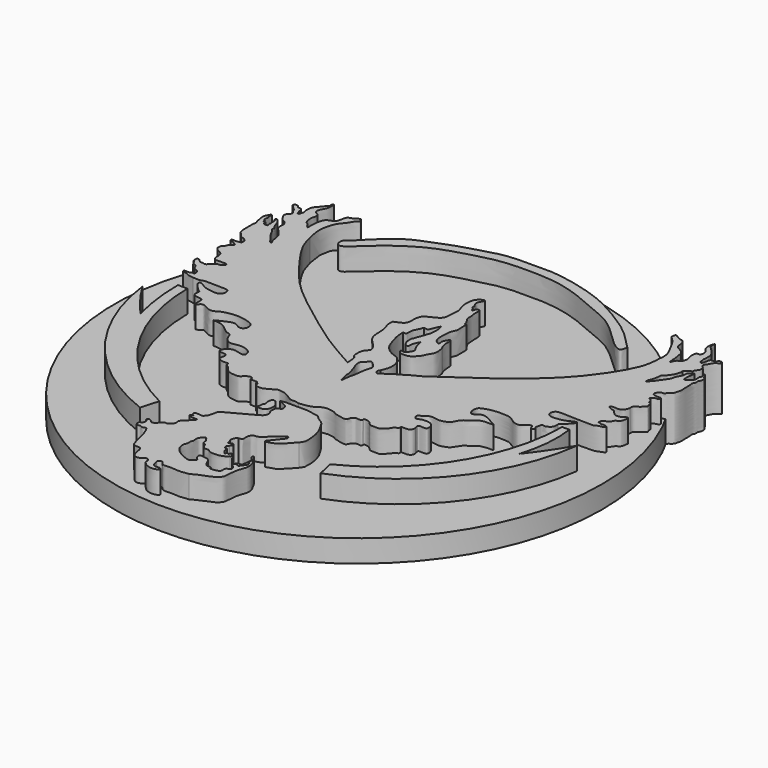
from build123d import *

# Parameters (mm, degrees)
F1_DEPTH = 10.16
F2_DEPTH = 10.16
F3_R     = 55.3641201476
F4_DEPTH = 5.08


with BuildPart() as f1:
    # F0 (on Top) → F1 (new body)
    with BuildSketch(Plane.XY):
        with BuildLine():
            add(Edge.make_bspline(
                [(-38.4339988232, 37.8163568676), (-40.3776892964, 36.5349947754), (-43.4388132675, 33.8198999387), (-45.1989802193, 31.6847162779), (-47.2682613555, 30.4657304543), (-46.3814242786, 27.8555501442), (-43.4019740855, 30.2386878564), (-39.710133046, 33.9622172552), (-33.2224238213, 38.1348936985), (-27.4582159472, 39.8824540183), (-20.6977212777, 41.8785343294), (-13.9519678519, 42.1607154766), (-7.111448046, 41.8507060169), (-1.2541898469, 40.1347538194), (3.8892959818, 37.7462480969), (9.0731299211, 35.8347678091), (13.3012948281, 31.7604990804), (15.8394430151, 29.1906952303), (18.03525943, 28.082935927), (18.1748118436, 29.369360897), (18.2424709201, 29.9906991422)],
                knots=[0, 0, 0, 0, 0.0668596402, 0.1107523169, 0.1484714431, 0.1817658099, 0.2255335492, 0.2880295411, 0.3602735162, 0.4251319675, 0.4940634431, 0.5624882713, 0.6309131089, 0.6954921303, 0.757679825, 0.8193358192, 0.8826101886, 0.9337790209, 0.9679766181, 1, 1, 1, 1], degree=3))
            add(Edge.make_bspline(
                [(18.2424709201, 29.9906991422), (17.8141330334, 30.408830657), (16.7527281886, 31.444944504), (13.7938974328, 34.6880180437), (8.1566619701, 38.3094929816), (2.3201213867, 41.540400936), (-5.2655643523, 43.6488415852), (-8.6701240685, 44.0560494137), (-10.1752104238, 44.2360676825)],
                knots=[0, 0, 0, 0, 0.1023686336, 0.2536655455, 0.4431101332, 0.6350204958, 0.8386500113, 1, 1, 1, 1], degree=3))
            add(Edge.make_bspline(
                [(-10.1752104238, 44.2360676825), (-12.8326389355, 44.270788298), (-17.4404864765, 44.3295572757), (-21.5624899491, 43.9615039159), (-26.1251831518, 42.5325010883), (-30.4255647938, 41.3167770675), (-33.883752839, 39.8140886356), (-36.8898562382, 38.7556979506), (-38.4339988232, 37.8163568676)],
                knots=[0, 0, 0, 0, 0.2056139755, 0.3591740502, 0.5235485789, 0.6838045267, 0.8302551077, 1, 1, 1, 1], degree=3))
        make_face()
    extrude(amount=F1_DEPTH)


with BuildPart() as f1b:
    # F0 (on Top) → F1, piece 2 (new body)
    with BuildSketch(Plane.XY):
        with BuildLine():
            ThreePointArc((28.3296834677, -1.1114582885), (21.9588448441, -22.8278664884), (5.1477458328, -37.9796624184))
            Line((5.1477458328, -37.9796624184), (5.9756720439, -41.7442247272))
            ThreePointArc((5.9756720439, -41.7442247272), (25.4686658342, -27.3806945741), (34.870300442, -5.0670872442))
            ThreePointArc((34.870300442, -5.0670872442), (31.998811419, -9.5991312123), (28.8264378905, -13.9258988202))
            ThreePointArc((28.8264378905, -13.9258988202), (30.1203901127, -7.5832981016), (29.9855358899, -1.1114582885))
            Line((29.9855358899, -1.1114582885), (28.3296834677, -1.1114582885))
        make_face()
    extrude(amount=F1_DEPTH)


with BuildPart() as f1c:
    # F0 (on Top) → F1, piece 3 (new body)
    with BuildSketch(Plane.XY):
        with BuildLine():
            add(Edge.make_bspline(
                [(-16.9677510858, -24.5513580739), (-16.7256834243, -24.4821800398), (-16.1652979406, -24.3220332201), (-14.7836189898, -24.343620097), (-12.6079063976, -24.3625652298), (-10.7965708244, -24.2642481241), (-9.235040639, -24.7639249566), (-8.1216758077, -24.7093805359), (-7.4935649662, -25.7020488651), (-5.9392442403, -26.3219035671), (-5.2102442975, -27.917648712), (-4.5029768556, -28.9924757201), (-3.9662952345, -30.6812746558), (-3.8195125267, -32.1406451632), (-3.6614700919, -34.0324624627), (-4.2100632963, -34.6319537439), (-4.4505232945, -34.8947234452)],
                knots=[0, 0, 0, 0, 0.0528153057, 0.1222671813, 0.2105244587, 0.291481933, 0.3668079203, 0.4261096568, 0.4867404698, 0.5621913496, 0.6389934812, 0.7071670237, 0.7845117462, 0.8586098391, 0.9380257036, 1, 1, 1, 1], degree=3))
            add(Edge.make_bspline(
                [(-22.5055478513, -34.390475601), (-21.9259403188, -34.0505378971), (-20.7189644235, -33.3426509366), (-18.6454880172, -32.3237794617), (-16.5514853718, -31.1531230316), (-15.5936887276, -30.6211560465), (-15.3322225029, -29.2716267624), (-15.9210427531, -28.8127335327), (-15.8293916152, -28.0452724683), (-15.8519796377, -27.1114892846), (-15.3011185582, -26.9889440966), (-14.6140773099, -26.6696913969), (-14.7809401703, -26.072075705), (-15.0705441145, -25.4008451103), (-15.8150471474, -25.0690802668), (-16.359271726, -24.8472614015), (-16.7611534973, -24.6518264184), (-16.9677510858, -24.5513580739)],
                knots=[0, 0, 0, 0, 0.0968855866, 0.2017547409, 0.3062678019, 0.3761599213, 0.4491018108, 0.5030952176, 0.5617460731, 0.6236759501, 0.6712721363, 0.7261272911, 0.7746796049, 0.832290549, 0.8920056908, 0.9444827672, 1, 1, 1, 1], degree=3))
            add(Edge.make_bspline(
                [(-26.231309399, -41.9427230954), (-26.1794664364, -41.7719131164), (-26.0512405981, -41.3494401007), (-25.0522160588, -40.5249387809), (-24.3386830564, -39.8691158598), (-23.8115959247, -39.1083890267), (-24.9532103468, -39.3424884377), (-25.5729615743, -39.0643236309), (-25.9995645417, -39.1608011011), (-26.204653708, -38.4924400788), (-25.1929828294, -38.478076012), (-25.9578219493, -38.3589435062), (-25.9803618013, -38.0725478094), (-26.1184276665, -37.4612283238), (-25.1667432362, -37.5119141629), (-24.3553437506, -37.578429159), (-23.9202085009, -37.6626431957), (-23.8747140177, -37.1944214738), (-23.4666182194, -36.9341756534), (-23.3189351114, -36.3070238564), (-23.1166480867, -35.6577637715), (-23.1112828619, -34.920560879), (-22.7112144825, -34.5704567008), (-22.5055478513, -34.390475601)],
                knots=[0, 0, 0, 0, 0.0468606991, 0.1159029523, 0.1806528883, 0.2254826523, 0.2813658817, 0.3341958213, 0.3707218661, 0.4111370699, 0.4562241953, 0.4944466264, 0.5278592271, 0.5689225269, 0.6227289098, 0.6814369735, 0.7167886129, 0.7537850262, 0.7953318701, 0.8436030607, 0.8949234566, 0.9459823875, 1, 1, 1, 1], degree=3))
            add(Edge.make_bspline(
                [(-26.9771926105, -53.5281673074), (-27.2904116425, -52.1829647833), (-27.8354985831, -49.8419437939), (-28.9047144408, -47.2120177249), (-29.4278921215, -47.6788043846), (-30.0685420899, -47.7334429906), (-30.2940893578, -47.3929876506), (-30.8440961772, -47.5589271277), (-31.2548479782, -47.6257107049), (-31.2354068332, -47.2735642737), (-31.4859604542, -47.0334377663), (-31.3801709377, -46.7515255689), (-31.4771736531, -46.4095666206), (-31.2436708212, -46.4021947), (-31.011613696, -46.4804211536), (-30.8634652488, -46.1636356398), (-30.7379304053, -46.1090136058), (-30.7090235419, -45.6426458975), (-30.6346845674, -45.0771151211), (-31.1806203221, -45.0957811047), (-31.0964682486, -44.3966953152), (-30.5624046689, -44.5643332988), (-30.0335186658, -44.8077926069), (-29.6664240229, -45.3721994941), (-28.8144658682, -44.8585942501), (-28.5599555229, -44.4914079264), (-28.1239387046, -43.9059311473), (-27.6746812945, -43.7472520307), (-27.029246442, -43.8762830859), (-26.5028861605, -43.197157612), (-26.1443403081, -42.8800023468), (-26.1570264533, -42.2276980028), (-26.2096483941, -42.025822154), (-26.231309399, -41.9427230954)],
                knots=[0, 0, 0, 0, 0.0909033619, 0.1581967581, 0.1872970966, 0.2215585782, 0.2474407242, 0.2804358885, 0.3062492454, 0.3292809787, 0.3543239279, 0.3783007145, 0.4022677612, 0.4204053642, 0.4412995114, 0.4655585057, 0.4811868872, 0.511297348, 0.5424325361, 0.5694484006, 0.5994618255, 0.6286403616, 0.6637706855, 0.6967032068, 0.7371432747, 0.7689146312, 0.8059043295, 0.8360533833, 0.8703378185, 0.9100626656, 0.9412021579, 0.9757967812, 1, 1, 1, 1], degree=3))
            add(Edge.make_bspline(
                [(-20.9622289985, -57.716358453), (-20.9940106039, -57.2651068123), (-21.0516010933, -56.447407312), (-22.124108515, -56.5414341853), (-22.4401063808, -57.2300135846), (-24.2688775072, -57.4196852814), (-24.6162129295, -55.4304841098), (-24.9460906879, -53.8259896786), (-26.3396652942, -54.167925755), (-26.7742181614, -53.7318520988), (-26.9771926105, -53.5281673074)],
                knots=[0, 0, 0, 0, 0.125756068, 0.2278787813, 0.3278672475, 0.4664722825, 0.6264317097, 0.7667036772, 0.8910300768, 1, 1, 1, 1], degree=3))
            add(Edge.make_bspline(
                [(-12.0712993667, -56.5152578056), (-12.7493936044, -56.6295703005), (-14.1237109247, -56.8612514342), (-16.1858497517, -56.4987947675), (-18.1777852045, -56.8882002364), (-18.6267076864, -55.4750181284), (-19.6833871052, -56.040200466), (-19.517722557, -56.5009885586), (-19.1391340004, -58.3367545726), (-17.6808140326, -57.731282123), (-16.860959846, -58.4258628207), (-18.4391241733, -59.1718949329), (-20.2898968367, -58.5915292695), (-20.7620721694, -57.9769014191), (-20.9622289985, -57.716358453)],
                knots=[0, 0, 0, 0, 0.1061933614, 0.2152258015, 0.313851804, 0.3896689792, 0.4557070212, 0.5056410018, 0.5966164576, 0.6796548057, 0.7373465413, 0.8210196444, 0.9241295807, 1, 1, 1, 1], degree=3))
            add(Edge.make_bspline(
                [(-18.6901520938, -50.8731864393), (-18.2250603004, -51.2113316134), (-17.3537289618, -51.8448334113), (-16.0828782386, -52.1989512747), (-15.2732204468, -52.47287834), (-14.0786614938, -51.3281023981), (-14.8796717674, -50.9889629162), (-15.4213045397, -49.4379472496), (-13.7780972027, -49.8516931938), (-13.0198678083, -49.8750937118), (-12.3540198093, -50.8712239402), (-12.1211868744, -51.7237818613), (-11.4198051638, -52.2705774023), (-10.5149189548, -51.9492873872), (-10.7602495431, -52.6881546449), (-9.3255101033, -52.5440197581), (-8.1486671478, -52.2033372076), (-8.5402887424, -50.6671022245), (-7.3345695029, -50.6200842936), (-7.3648357078, -49.6419480924), (-8.0291574769, -49.3227063851), (-8.5999063873, -48.585002508), (-7.7755432562, -48.2572130335), (-7.0193120942, -48.9484661499), (-6.9588836312, -48.0277235349), (-6.1273259776, -47.6446762184), (-6.0680808625, -46.5787323534), (-6.9934236024, -46.3403453634), (-6.1837791819, -45.6199933483), (-7.6395276348, -44.753535211), (-7.3435095655, -43.8025659858), (-6.5640552282, -45.0858518438), (-5.6055039784, -46.5742573026), (-5.5136890207, -48.2714689857), (-6.4220104344, -50.0482570837), (-6.4997083315, -52.4557682302), (-6.6337639731, -53.883545983), (-8.5998715213, -55.0730106395), (-10.2125303956, -55.53117938), (-11.4877454779, -56.1985231624), (-11.9034585019, -56.4241590786), (-12.0712993667, -56.5152578056)],
                knots=[0, 0, 0, 0, 0.0327909925, 0.0614326457, 0.0843446193, 0.1122801907, 0.1326685665, 0.1592610519, 0.1868977959, 0.2097865402, 0.2360156409, 0.2601429026, 0.2829593096, 0.3038495752, 0.3188906288, 0.3465005671, 0.37315175, 0.4001342324, 0.4234373585, 0.4444687778, 0.4665626336, 0.4876551678, 0.5072587528, 0.528972298, 0.5482121835, 0.5720055441, 0.5952223763, 0.6152317394, 0.6346038596, 0.6646880614, 0.6822516525, 0.7084308903, 0.7435788646, 0.7753179277, 0.8110108254, 0.8500815365, 0.8793502778, 0.916054146, 0.9500085639, 0.9798163507, 1, 1, 1, 1], degree=3))
            add(Edge.make_bspline(
                [(-10.6587931514, -46.6785617173), (-10.8635270992, -46.886411231), (-11.3269579996, -47.3568944523), (-12.6367521866, -47.7503959709), (-14.6661988628, -47.7283628095), (-14.9307405353, -47.1379809006), (-15.587708552, -47.0802588979), (-16.0650433064, -47.2181035102), (-16.5430461175, -46.6383479232), (-16.8911729594, -46.1693765723), (-16.8545790521, -45.7672708134), (-17.5343681361, -45.7167704548), (-17.6967493612, -45.165503417), (-17.6322821726, -44.6607620455), (-18.2185792059, -44.1919181968), (-18.1677240334, -43.6090224646), (-18.9369523108, -44.1109424358), (-19.5833851043, -44.79175125), (-19.4362316795, -45.5592943927), (-19.4265306191, -46.2781674795), (-19.7082278346, -46.6013840635), (-19.5667226668, -47.6863146408), (-20.0105690508, -48.0488033747), (-19.90516408, -49.703706402), (-19.1062300064, -50.4727008323), (-18.6901520938, -50.8731864393)],
                knots=[0, 0, 0, 0, 0.0478082612, 0.1082176443, 0.1779063426, 0.2146642285, 0.2533004876, 0.2874426533, 0.3295266129, 0.3685827028, 0.3964402805, 0.4338799673, 0.4697945662, 0.5050191127, 0.5474975527, 0.5776980102, 0.6192765657, 0.668706555, 0.7123174915, 0.7537778216, 0.7863276831, 0.836393555, 0.8730753788, 0.9338987619, 1, 1, 1, 1], degree=3))
            add(Edge.make_bspline(
                [(-13.8497008011, -40.3151884675), (-13.9666380743, -40.4017415398), (-14.2325429571, -40.5985554718), (-14.5559454424, -41.2328294146), (-14.5824055623, -42.0797889253), (-14.0970981384, -42.1034918907), (-14.3539283978, -43.0717812167), (-13.5658390206, -42.6154715779), (-12.9937447588, -42.5290467211), (-12.8940141695, -43.4631833459), (-13.3776245222, -43.2100732068), (-13.1188447765, -43.9522844857), (-13.5541340128, -43.7253786325), (-13.600378754, -44.2544597954), (-13.5253164947, -44.7455708776), (-13.0303636652, -44.6305137642), (-12.6667559179, -44.8459457857), (-12.9248373064, -45.729313477), (-12.337387765, -45.9030213897), (-12.0801345541, -46.6639734723), (-11.7500406528, -45.79771422), (-11.456239961, -46.3708890058), (-10.9698667067, -45.359783), (-10.9496954458, -46.0945687662), (-10.5057155668, -46.0486761811), (-10.4082974123, -46.5503901899), (-10.5814288812, -46.6389766261), (-10.6587931514, -46.6785617173)],
                knots=[0, 0, 0, 0, 0.0401509526, 0.0912996689, 0.1419571028, 0.1754094704, 0.2220730175, 0.2686298994, 0.3108094826, 0.3574730297, 0.3857473753, 0.4262792981, 0.4544092326, 0.4931195944, 0.5320698283, 0.5701703842, 0.6043756027, 0.6556527339, 0.6998295744, 0.7413613998, 0.7834109177, 0.8150481175, 0.8627694576, 0.8979069629, 0.9334600484, 0.9702664407, 1, 1, 1, 1], degree=3))
            add(Edge.make_bspline(
                [(-4.4505232945, -34.8947234452), (-4.9507640677, -35.4464675067), (-5.9248899768, -36.5208864954), (-6.997557859, -37.8230520634), (-10.050521006, -38.7208985221), (-8.6389909124, -37.1588717516), (-7.7138375546, -35.8043184859), (-6.8294427645, -34.9862826352), (-7.2629678047, -34.2047864512), (-8.3673787201, -34.9329868996), (-10.171459098, -36.8174674985), (-11.5093494092, -37.9438799896), (-12.5526042936, -37.6531204088), (-13.1637765938, -38.9988990986), (-12.7600472062, -40.2959565151), (-13.5025949725, -40.3090621877), (-13.8497008011, -40.3151884675)],
                knots=[0, 0, 0, 0, 0.0886799871, 0.1726877889, 0.2608507845, 0.3260190157, 0.4102249389, 0.4724048651, 0.5162846431, 0.5781901774, 0.6796395885, 0.7577030776, 0.8128946044, 0.8808954204, 0.9443242635, 1, 1, 1, 1], degree=3))
        make_face()
    extrude(amount=F1_DEPTH)


with BuildPart() as f1d:
    # F0 (on Top) → F1, piece 4 (new body)
    with BuildSketch(Plane.XY):
        with BuildLine():
            add(Edge.make_bspline(
                [(-18.2506423444, -25.0749997795), (-18.1274044818, -24.9866210706), (-17.7372615676, -25.0490418709), (-17.2778145772, -25.3504363014), (-16.8666657328, -25.9999192655), (-16.5880790984, -26.3871950157), (-16.3949385176, -27.5819302408), (-16.845514393, -28.4299032771), (-17.2288009915, -28.8501613979), (-18.2008410285, -28.9667204973), (-19.0093898141, -28.8779515366), (-18.5290154176, -28.0901185387), (-18.7221607056, -27.4186664462), (-18.2330715439, -26.9874234197), (-18.5444617547, -26.2777623363), (-18.5100466403, -25.6995174157), (-18.3936348795, -25.1775453394), (-18.2506423444, -25.0749997795)],
                knots=[0, 0, 0, 0, 0.0558298724, 0.1170354669, 0.1865450272, 0.2435943279, 0.330616603, 0.4091921431, 0.4683067793, 0.5494010315, 0.6108988649, 0.6782508715, 0.7447590423, 0.8037918518, 0.8707540407, 0.9352207608, 1, 1, 1, 1], degree=3))
        make_face()
    extrude(amount=F1_DEPTH)


with BuildPart() as f1e:
    # F0 (on Top) → F1, piece 5 (new body)
    with BuildSketch(Plane.XY):
        with BuildLine():
            add(Edge.make_bspline(
                [(-16.8645642698, -5.520043429), (-16.8901329775, -5.2359622568), (-16.9463157343, -4.6117436374), (-17.0361507413, -3.1519554938), (-17.7108247589, -2.8376420104), (-17.7852414032, -1.4689009073), (-17.5346312587, 0.0844993321), (-16.3751440954, 0.6871318957), (-17.2187440528, 2.3350999393), (-18.5262626691, 3.4892288988), (-19.3929748031, 4.4935721312), (-19.7685458929, 5.9866931281), (-19.7384534158, 7.5248848306), (-19.9259606118, 9.1344560926), (-20.5279578718, 10.2677189196), (-20.4470927827, 11.2201422151), (-20.405350253, 11.7117827758)],
                knots=[0, 0, 0, 0, 0.0606283276, 0.133220131, 0.1820477962, 0.2522057423, 0.3299423507, 0.3921717653, 0.4689539906, 0.5533715348, 0.6241288831, 0.6996450389, 0.7778293529, 0.8564007325, 0.92587411, 1, 1, 1, 1], degree=3))
            add(Edge.make_bspline(
                [(-52.0574450493, 27.8376024216), (-51.8040302595, 26.8173723951), (-51.2163186536, 24.4512870221), (-47.945431617, 19.5775374826), (-42.3974763198, 12.1992258136), (-34.9349582293, 6.4374371833), (-26.2793050468, -0.0487255694), (-21.6626759759, -2.8312436721), (-18.4611972258, -4.6253109661), (-16.8645642698, -5.520043429)],
                knots=[0, 0, 0, 0, 0.0993678639, 0.2304508229, 0.3960239687, 0.5675796854, 0.7461321333, 0.8733916936, 1, 1, 1, 1], degree=3))
            add(Edge.make_bspline(
                [(-54.7654815018, 30.552232638), (-54.7854907508, 31.0739918196), (-54.8274878122, 32.1691030073), (-54.5197462951, 34.1905682518), (-53.7865112274, 35.0743807001), (-52.2913875565, 35.2551152241), (-52.058681307, 36.5836555361), (-51.8058372767, 38.1085532107), (-50.6353340027, 38.0851784418), (-49.2621381334, 39.3378980518), (-49.2931000522, 38.4351622307), (-48.809326309, 38.1376075067), (-49.8120160183, 37.5344642515), (-50.3051102963, 36.2693623487), (-51.4395030187, 35.2135824605), (-52.232511626, 33.3989828396), (-52.6280818192, 31.2414371681), (-52.4048913474, 29.605132096), (-52.1749181667, 28.4352119577), (-52.0574450493, 27.8376024216)],
                knots=[0, 0, 0, 0, 0.0657283905, 0.1379561651, 0.1908566264, 0.2486790504, 0.3057066469, 0.3649773818, 0.41861489, 0.478988609, 0.515449969, 0.546996258, 0.5950937686, 0.6556226667, 0.7184863265, 0.7903474262, 0.8658618495, 0.9314805898, 1, 1, 1, 1], degree=3))
            add(Edge.make_bspline(
                [(-62.2118934989, 35.5500467122), (-62.1964625512, 35.6872215646), (-62.1648794291, 35.9679826818), (-61.727195536, 36.151728379), (-60.9851801432, 35.8233669891), (-61.2540732904, 35.4415514221), (-60.3164536711, 35.5569036516), (-59.7437300382, 35.059134312), (-59.9789680914, 34.3740726536), (-59.5115571609, 34.1391143781), (-59.705101711, 33.6157970819), (-59.0724105195, 33.6093552109), (-59.2040518081, 34.2130375113), (-58.8638123348, 34.5319121504), (-59.1259526516, 35.0460417342), (-59.1681982379, 36.5395921672), (-58.7400386776, 37.4211844288), (-57.9115783097, 38.2053291849), (-57.4673374838, 38.903498425), (-56.7596438557, 39.3777573672), (-57.0763359762, 40.1751306621), (-56.4335780123, 40.5074581172), (-56.581927353, 39.3399774924), (-56.6271079384, 38.2805871993), (-57.3665826944, 37.2564822252), (-57.5895013628, 36.2610891349), (-57.0675769, 35.7644756841), (-56.4563229889, 35.7008217897), (-56.2416469628, 34.3696023782), (-56.5730847922, 34.141361128), (-56.4919693881, 32.9022868844), (-56.4071653043, 32.3544099022), (-55.964693112, 31.6466613688), (-55.5435139108, 31.6860265061), (-55.2723049751, 30.8266489361), (-54.9249399097, 30.6385703636), (-54.7654815018, 30.552232638)],
                knots=[0, 0, 0, 0, 0.0224888245, 0.0460287536, 0.0757331999, 0.0921965553, 0.1231258223, 0.1530626503, 0.1808831059, 0.2039528356, 0.226614165, 0.248155141, 0.2735619363, 0.2961905238, 0.3219062773, 0.3657033207, 0.4019810604, 0.4400116837, 0.4734917327, 0.5045790405, 0.5350511221, 0.5564225968, 0.5902788081, 0.6294687819, 0.6698730003, 0.7048105639, 0.7328939335, 0.7596847003, 0.7983326215, 0.8206879989, 0.8592217064, 0.8884724464, 0.9193424938, 0.9403879815, 0.9726350215, 1, 1, 1, 1], degree=3))
            add(Edge.make_bspline(
                [(-63.3470118046, 29.5983385295), (-63.2401709146, 29.8558807254), (-63.0709242297, 30.2638533927), (-62.5756726403, 30.463039179), (-62.9045030164, 29.5152403725), (-62.4812165758, 29.0988153673), (-62.9136997256, 28.1744331608), (-62.2223762626, 27.9173747263), (-62.6130958871, 27.3328614169), (-61.7337083094, 27.5439966332), (-61.9883089735, 27.110873109), (-61.5927546568, 26.6369875744), (-60.6903589543, 26.5739510377), (-61.0024384761, 27.3511054621), (-60.8099251965, 27.8478131692), (-61.0087980538, 28.2075728247), (-60.858480248, 29.1372239732), (-61.4062624341, 29.1707407224), (-61.1150550178, 29.8633709205), (-60.2737405991, 29.0030905731), (-59.9808833898, 28.0745537786), (-59.6631154773, 27.088885239), (-59.1325066006, 26.6936514709), (-59.4448871042, 26.0182524843), (-58.6768728862, 25.4486925613), (-58.3400440704, 24.35533948), (-57.3877609309, 23.258434713), (-56.8064206325, 22.477173263), (-56.2922982036, 21.7043757322), (-56.059782912, 22.2579733315), (-56.5853994302, 22.5317700987), (-56.5433884957, 23.4194755154), (-56.8515746687, 24.1494598937), (-56.8326351444, 25.0628419074), (-57.4788836491, 25.480552391), (-57.9833973913, 26.449468062), (-58.5193636199, 26.5040185378), (-59.0009812027, 27.8916646051), (-58.7064117884, 28.5863536152), (-59.1469797169, 29.7541795676), (-60.231904076, 29.9992855464), (-60.6787044133, 30.8592384986), (-61.2249176775, 31.7204677198), (-60.6859132403, 32.4801765962), (-60.0771110469, 33.0552691626), (-60.7307963819, 33.6845190662), (-60.8759093022, 34.3367143669), (-61.4313736465, 34.815867935), (-61.8876337575, 35.2224052553), (-62.1096392347, 35.4467260348), (-62.2118934989, 35.5500467122)],
                knots=[0, 0, 0, 0, 0.0217580607, 0.0344669503, 0.0558728381, 0.0747784714, 0.0972436214, 0.1151301931, 0.1301560184, 0.1481491532, 0.1610925294, 0.1799410391, 0.1998402908, 0.2193609538, 0.237196421, 0.2531784449, 0.2756435949, 0.2902609707, 0.3056922189, 0.3293730472, 0.3555654029, 0.3806243879, 0.3993492936, 0.4180742088, 0.4406958899, 0.4675679079, 0.4974424254, 0.5236216828, 0.5439608034, 0.5577353013, 0.5751881499, 0.5977897559, 0.6205306809, 0.6431322869, 0.6646777234, 0.6897881221, 0.706984504, 0.7353807408, 0.7575504798, 0.783391787, 0.8085889757, 0.8328353973, 0.8567960874, 0.8798462502, 0.9006077468, 0.9219889574, 0.9425399736, 0.9635559702, 0.9832141193, 1, 1, 1, 1], degree=3))
            add(Edge.make_bspline(
                [(-62.9924535751, 21.9058506191), (-63.0359836807, 21.9878510025), (-63.1659905682, 22.2327531106), (-63.159197377, 23.5329721036), (-63.2309246353, 25.4175243848), (-63.0070242015, 26.4847453594), (-63.3079674165, 26.6996632495), (-63.3517015677, 27.2063691406), (-63.465409795, 27.851270096), (-63.582425017, 28.2255141972), (-63.6210259139, 29.0706895869), (-63.4335931104, 29.4316152372), (-63.3470118046, 29.5983385295)],
                knots=[0, 0, 0, 0, 0.0668454118, 0.1996403137, 0.36907731, 0.4856100648, 0.548521912, 0.6312229859, 0.7267277223, 0.8026833979, 0.9088530463, 1, 1, 1, 1], degree=3))
            add(Edge.make_bspline(
                [(-61.8908368051, 20.5466300249), (-61.9901176092, 20.6582843141), (-62.2038702735, 20.898677228), (-62.5817190284, 21.444883813), (-62.9338155536, 21.4973313396), (-62.972186691, 21.7646553213), (-62.9924535751, 21.9058506191)],
                knots=[0, 0, 0, 0, 0.2619254443, 0.5639283653, 0.7696754928, 1, 1, 1, 1], degree=3))
            add(Edge.make_bspline(
                [(-61.6110116243, 16.0841420293), (-61.633170487, 16.2020151186), (-61.6814078337, 16.4586115499), (-61.2850389645, 16.8387566458), (-60.892254043, 16.8977683034), (-60.6730023654, 17.3794361826), (-61.1243664783, 17.6283563045), (-61.4413800901, 17.6670698803), (-61.58298237, 18.0099121568), (-62.0660535204, 17.7908950386), (-62.5506509366, 18.1678812828), (-62.3510323604, 18.630643664), (-61.5730713011, 18.4215747339), (-61.0030865478, 18.6490099888), (-60.2957620576, 18.5823159653), (-60.2292159592, 19.3543138911), (-60.4978677571, 19.8136598213), (-61.0648000425, 20.2245692673), (-61.4878864282, 20.2578099283), (-61.7531790876, 20.4479620063), (-61.8908368051, 20.5466300249)],
                knots=[0, 0, 0, 0, 0.0483106236, 0.105166783, 0.1562491288, 0.2070812652, 0.2603747051, 0.3061432504, 0.3484263155, 0.402454204, 0.4601285616, 0.5063105667, 0.5746319257, 0.6404547987, 0.7019070611, 0.7648902377, 0.8250681532, 0.8912294516, 0.9435600463, 1, 1, 1, 1], degree=3))
            add(Edge.make_bspline(
                [(-60.5396553874, 12.9524311051), (-60.6852143475, 13.1150595096), (-60.9945535509, 13.4606743798), (-61.8290727902, 13.7192919442), (-62.1433094859, 14.2269192958), (-62.4256303538, 14.3628976344), (-62.3752261568, 14.6691556297), (-62.4212532131, 15.0471724216), (-62.2802115606, 15.4739799876), (-61.8791338211, 15.8489301085), (-61.6938654642, 16.0114579656), (-61.6110116243, 16.0841420293)],
                knots=[0, 0, 0, 0, 0.1335259638, 0.2837669027, 0.4071160645, 0.4903047609, 0.5742793538, 0.6751265739, 0.7829690671, 0.9029416223, 1, 1, 1, 1], degree=3))
            add(Edge.make_bspline(
                [(-62.2566007078, 7.4995243922), (-62.2907509688, 7.6178887265), (-62.3588193786, 7.8538128967), (-62.7440939578, 8.0229369941), (-62.6983870462, 8.4547744221), (-62.7256102718, 9.0569244139), (-61.9807026769, 8.9499577474), (-61.6469627685, 8.4100154392), (-61.093569136, 8.1929269059), (-60.7128408087, 8.3939613356), (-60.1865922754, 7.9860288778), (-59.6062565781, 8.6679205339), (-58.8900532555, 9.4377837682), (-58.3639797815, 9.6088250342), (-57.8716617125, 9.5215879341), (-57.3016866948, 9.9786308379), (-56.8942718793, 10.6300676684), (-58.0781019893, 10.6320352004), (-58.9833972965, 10.6552155227), (-59.7236382187, 10.5794115506), (-60.152769289, 10.8742878964), (-60.3598541244, 11.3245394329), (-60.3697176114, 11.952568702), (-60.3541993253, 12.3068704011), (-60.4013639962, 12.565350536), (-60.4898890212, 12.813133979), (-60.5396553874, 12.9524311051)],
                knots=[0, 0, 0, 0, 0.0337104428, 0.0671917625, 0.1033964129, 0.1424441484, 0.1840121964, 0.2295743903, 0.2707366205, 0.3056401871, 0.3457030118, 0.3955652093, 0.454636961, 0.495065375, 0.5330912242, 0.5817199278, 0.621276189, 0.6744865555, 0.7319742997, 0.7792473894, 0.8177848139, 0.8570401279, 0.9018328314, 0.9352563276, 0.9636028647, 1, 1, 1, 1], degree=3))
            add(Edge.make_bspline(
                [(-58.6782768369, 2.818579087), (-58.9498509273, 2.8453527153), (-59.4633642098, 2.8959783612), (-60.0924402614, 3.1341035966), (-60.4465425692, 3.3563685631), (-61.2399148549, 3.4815129254), (-61.6372123512, 3.6011657165), (-61.5203236226, 4.0080486294), (-60.8609597253, 3.9848648377), (-60.1501737369, 3.8935162446), (-59.9021682882, 4.2960920958), (-59.3121348389, 3.9763484582), (-59.3954934659, 4.8901258044), (-59.6740263137, 5.3301740785), (-60.4745071096, 5.6350248389), (-60.8132347317, 5.9220800414), (-60.9276290832, 6.3921805069), (-61.2318851342, 6.8948524512), (-61.8903848606, 6.7119398274), (-61.9067692005, 7.1841146255), (-62.1265942343, 7.3630803334), (-62.2163169368, 7.4572458728), (-62.2566007078, 7.4995243922)],
                knots=[0, 0, 0, 0, 0.0641153897, 0.1212343349, 0.1679967888, 0.2323539535, 0.2742296567, 0.3107720678, 0.3669657972, 0.4266416602, 0.4701536818, 0.5154813313, 0.5731014216, 0.6267480502, 0.6912106271, 0.7378929585, 0.7869691426, 0.8384491226, 0.8895516065, 0.9317700926, 0.9693660814, 1, 1, 1, 1], degree=3))
            add(Edge.make_bspline(
                [(-54.2273372412, -2.234257292), (-54.3312010787, -2.0980637809), (-54.5459152484, -1.8165155797), (-54.4028364714, -1.2767240025), (-54.3958828672, -0.4968116173), (-54.9181199274, -0.3595103182), (-55.2609944104, 0.0077995497), (-55.6554260559, 0.4701069729), (-56.2923556001, 1.0204529125), (-56.5818994398, 1.5398886047), (-56.5858824279, 2.266204581), (-55.5306837232, 1.8433200861), (-54.8730350896, 1.2356480848), (-53.9947073, 1.0160987614), (-52.8045479477, 0.7415235268), (-50.9815289184, 0.6226126341), (-50.4255448942, 1.8336682854), (-50.7449995557, 3.0851905372), (-52.271381571, 2.9803020943), (-53.9480437239, 3.0306813094), (-56.2711486025, 3.1809481331), (-56.949461778, 2.7068965834), (-58.0324999686, 2.7768615088), (-58.6782768369, 2.818579087)],
                knots=[0, 0, 0, 0, 0.0343398017, 0.0709895011, 0.1119004626, 0.1451001985, 0.1794547827, 0.2182106136, 0.26321913, 0.3020605591, 0.3355907916, 0.3814971455, 0.4297925932, 0.4750219434, 0.5307739782, 0.5942531395, 0.6463196874, 0.6962239058, 0.7519370076, 0.8192369338, 0.8924494767, 0.9358714765, 1, 1, 1, 1], degree=3))
            add(Edge.make_bspline(
                [(-45.6152036786, -7.7210180461), (-44.8654163307, -7.3552941022), (-43.4857614034, -6.6823708172), (-41.618662575, -5.9770457326), (-40.436393068, -7.3032686192), (-39.0234574493, -6.7825584264), (-39.0041453237, -4.7176723674), (-40.9028265001, -4.1408975692), (-43.0031967154, -3.601849667), (-45.5816529943, -3.9525005882), (-46.9333167266, -4.4704599387), (-47.6740522128, -5.0258765197), (-49.086115145, -5.2337167924), (-50.8773961574, -3.481229317), (-52.0387825771, -5.6152593298), (-52.0788131271, -3.611955405), (-52.0854399011, -2.5327934848), (-53.2537033005, -2.6723375164), (-53.891861093, -2.3852086568), (-54.2273372412, -2.234257292)],
                knots=[0, 0, 0, 0, 0.07531635, 0.1392864396, 0.1979912981, 0.2489136592, 0.3096729297, 0.373094709, 0.4453841926, 0.5226720319, 0.5796812107, 0.6245271809, 0.6797509007, 0.748158282, 0.8016163882, 0.8557366334, 0.9036754118, 0.949622796, 1, 1, 1, 1], degree=3))
            add(Edge.make_bspline(
                [(-33.1087820232, -18.9998950809), (-33.5976769508, -19.0398167809), (-34.5168972375, -19.1148775649), (-35.8953397383, -18.5859472519), (-35.2661842682, -16.9792875918), (-35.9006959033, -16.3826224642), (-37.598172818, -16.6602502517), (-37.3431656406, -15.1129495537), (-36.0864166084, -14.3253197321), (-34.9346941018, -14.3457619704), (-32.7963184589, -15.1396605326), (-32.9297806834, -13.3054636587), (-34.507152733, -12.4634932334), (-36.0900931394, -12.3109980028), (-37.9633469635, -12.9917595179), (-39.4545810304, -11.6863123634), (-39.8062910501, -9.9241478053), (-40.9352003136, -10.0561752529), (-42.4159260494, -8.6016026095), (-43.7563657145, -7.8035444855), (-44.9816248799, -7.7491469112), (-45.6152036786, -7.7210180461)],
                knots=[0, 0, 0, 0, 0.0535564907, 0.1006969187, 0.1529070049, 0.1896161933, 0.2407865872, 0.286023728, 0.3382012149, 0.387701116, 0.4463282411, 0.4929972042, 0.5507133794, 0.6067729785, 0.6664615189, 0.7255079917, 0.7806789781, 0.8221741435, 0.8845701064, 0.9403114579, 1, 1, 1, 1], degree=3))
            add(Edge.make_bspline(
                [(-32.4323326349, -20.0201701373), (-32.7005831762, -19.8923442027), (-33.1993820301, -19.654658085), (-33.1374208932, -19.2068671687), (-33.1087820232, -18.9998950809)],
                knots=[0, 0, 0, 0, 0.5377930185, 1, 1, 1, 1], degree=3))
            add(Edge.make_bspline(
                [(-26.286913082, -20.8110008389), (-26.4306257362, -20.6998561996), (-26.7791369367, -20.4303242516), (-27.8922477943, -20.9481977892), (-28.4503313101, -21.7784329562), (-29.575591141, -21.7588580783), (-30.9112591872, -21.6720788981), (-31.8745050427, -20.8457050835), (-32.252825489, -20.2858246587), (-32.4323326349, -20.0201701373)],
                knots=[0, 0, 0, 0, 0.1049866699, 0.254598529, 0.3937252615, 0.5378547474, 0.7021240469, 0.8586625103, 1, 1, 1, 1], degree=3))
            add(Edge.make_bspline(
                [(-23.5335603356, -22.7188598365), (-23.7638547174, -22.6876036283), (-24.1922400407, -22.6294619545), (-24.1676757961, -22.1324683921), (-24.2045428346, -21.6468742983), (-24.7471927877, -21.897234935), (-24.621758259, -21.3928817858), (-24.9538924384, -21.3074921095), (-25.7729541649, -21.36564671), (-26.4628313584, -21.3549455316), (-26.343757282, -20.9867648443), (-26.286913082, -20.8110008389)],
                knots=[0, 0, 0, 0, 0.1272113828, 0.2366340374, 0.3366861624, 0.4341375692, 0.5274046699, 0.6115381432, 0.7678211151, 0.8891612401, 1, 1, 1, 1], degree=3))
            add(Edge.make_bspline(
                [(-13.9366751537, -23.1849681586), (-14.234030766, -23.0981965695), (-14.8295947164, -22.9244045566), (-15.8406127951, -23.1107987372), (-16.3610486038, -22.6547996835), (-17.3724289714, -22.0833144743), (-18.2913699217, -21.5089940469), (-19.4017936718, -21.4571081319), (-19.9173911387, -21.2906054245), (-20.7725186881, -21.9062156367), (-21.7058715614, -22.375206391), (-22.6657073252, -22.8687261966), (-23.2540696246, -22.7671240644), (-23.5335603356, -22.7188598365)],
                knots=[0, 0, 0, 0, 0.0915684751, 0.1833995408, 0.2593095112, 0.3604304242, 0.4607155099, 0.5578613738, 0.6245565103, 0.7173338125, 0.8169835725, 0.9130614054, 1, 1, 1, 1], degree=3))
            add(Edge.make_bspline(
                [(5.9296735562, -18.8878625631), (5.9848062439, -19.1161935999), (6.1021305562, -19.6020901341), (5.1347731971, -19.7533336714), (4.8655006993, -20.5366316597), (4.1637518658, -21.1666954278), (3.3302647118, -22.0181959174), (2.2761351256, -21.7570945176), (1.3129829305, -21.9528503459), (0.7735135433, -21.333067446), (0.2946743661, -20.7919130563), (-0.43902193, -20.6852795625), (-1.1398954109, -20.6284696589), (-0.8588303968, -21.156740339), (-1.3323712424, -21.4262130137), (-2.1710096655, -21.2611276918), (-2.6506603272, -21.2808738629), (-2.7465445568, -21.7008665163), (-3.1634285864, -21.5709860176), (-3.1532959104, -23.0327528431), (-4.90498254, -22.5813119184), (-6.2750260005, -22.3185629221), (-6.8916342669, -21.7520161125), (-8.4984266033, -21.538778068), (-9.667156763, -21.664703598), (-10.7704925666, -22.6853718936), (-12.5337201312, -23.1055336294), (-13.488310873, -23.1595820236), (-13.9366751537, -23.1849681586)],
                knots=[0, 0, 0, 0, 0.0322142671, 0.0685531015, 0.1049814115, 0.1457278326, 0.1893643947, 0.2313129617, 0.2710602322, 0.3068729904, 0.3417162798, 0.3784049599, 0.4077651018, 0.4329303331, 0.4596400603, 0.4988412352, 0.5259429212, 0.5494112024, 0.5701004756, 0.6112244939, 0.6615313956, 0.7116229648, 0.7487541117, 0.8004962391, 0.8453062211, 0.8950325772, 0.9506975702, 1, 1, 1, 1], degree=3))
            add(Edge.make_bspline(
                [(8.2397963852, -17.602680251), (8.2618130313, -17.7846172004), (8.308528623, -18.170656571), (7.8987926409, -18.8718944328), (6.8281386515, -18.9316119034), (6.2246357913, -18.9022252838), (5.9296735562, -18.8878625631)],
                knots=[0, 0, 0, 0, 0.2102637443, 0.4461440285, 0.7293026992, 1, 1, 1, 1], degree=3))
            add(Edge.make_bspline(
                [(27.0992107689, -0.7722591981), (27.1310536673, -1.1096625579), (27.1913508853, -1.748564323), (26.7422440007, -2.4007002092), (25.6096318761, -2.9607343891), (24.9169184177, -2.4657395738), (24.9087340903, -3.4527953588), (24.5065776621, -4.3072183696), (25.4132486136, -4.6370873118), (24.1902652431, -5.2540968895), (24.1114831076, -4.078861716), (23.2778560721, -3.9826661911), (22.3628447095, -5.2086267924), (21.1529961707, -5.42599847), (19.9838843997, -4.8293956402), (19.6027851875, -4.3888119564), (18.4258078044, -3.7936987204), (17.5637175145, -3.8082782503), (16.1560125725, -3.6774135247), (14.1561568336, -3.927625202), (12.9470169063, -4.3286810139), (11.9142077725, -4.8078005561), (11.9185474518, -6.0777514136), (12.0401591046, -6.6092576465), (12.5687568222, -7.4385704354), (13.7958542045, -6.7486197251), (14.2393061467, -6.1920596593), (15.7602527934, -6.4615605652), (16.957227972, -7.3535757746), (18.9344972371, -8.1931360099), (16.6483220091, -8.0176689814), (15.5083399354, -8.1749880959), (14.1273592154, -9.0991631961), (13.7168297597, -9.5910530652), (12.8736910157, -10.0438397892), (12.1905584013, -11.0977764457), (11.7655070676, -12.2060871886), (10.1968521023, -12.6994855525), (9.2645650873, -12.755712457), (8.0657779353, -12.4054386329), (6.9579531451, -12.6218233714), (6.4913151644, -13.4570095457), (5.2085965009, -13.4527039179), (5.8550134906, -15.0994511617), (6.9245622965, -14.3994182278), (8.1753110082, -14.3131405378), (9.6310741502, -14.6130878729), (10.0879604848, -15.8699513494), (10.0083717576, -16.7119199223), (8.8913141065, -16.6663179193), (7.8547745845, -16.4910356317), (8.1076191223, -17.2210547358), (8.2397963852, -17.602680251)],
                knots=[0, 0, 0, 0, 0.0191787064, 0.0363165008, 0.0577883998, 0.0722349868, 0.0892582237, 0.1076450336, 0.1217316794, 0.1385937073, 0.1566641296, 0.1717337742, 0.1953323344, 0.2167245874, 0.2383617678, 0.2538231699, 0.2756387144, 0.2940255184, 0.3172992533, 0.3453982321, 0.3679326143, 0.3876414011, 0.4084495523, 0.4236449049, 0.4406857792, 0.4621576711, 0.4785656071, 0.5011379616, 0.5276274349, 0.5494681271, 0.5727418464, 0.5961796912, 0.6205844703, 0.6364318526, 0.6550658861, 0.6770144606, 0.6981160887, 0.7223206324, 0.7416547369, 0.7633943748, 0.7834684053, 0.8020211249, 0.8207487038, 0.8412301618, 0.860742586, 0.8832617383, 0.9063111148, 0.9281266716, 0.9439079816, 0.9637519292, 0.9810509223, 1, 1, 1, 1], degree=3))
            add(Edge.make_bspline(
                [(32.2207137942, 4.1695130058), (32.3749754431, 4.2539884975), (32.6596848851, 4.4098987336), (32.8666471062, 4.0159840481), (33.4846772962, 4.148120848), (34.1787507345, 4.1288783516), (34.5517939626, 3.6719300012), (33.5993434901, 3.2794823543), (32.8319850079, 3.2343228892), (32.3521913168, 2.7797233702), (31.2678335797, 2.842819025), (29.4550139808, 2.8030062069), (28.0196145141, 2.9751738452), (26.7842049736, 2.9590140488), (25.4942445398, 3.001282619), (24.2686528744, 2.9748397612), (23.5551564867, 2.737775976), (23.1749970784, 1.7107869251), (23.6389003283, 0.9617278034), (24.7198421849, 0.6679067997), (26.0105720917, 0.84946684), (27.169804264, 1.0569105097), (28.0473890615, 1.6058061234), (28.7792680521, 1.7883219754), (29.2448956148, 2.1820755777), (29.3152919901, 1.2899092105), (28.3821482162, 0.6590225858), (28.0609313281, -0.0663380466), (27.2197663567, -0.3192071879), (27.1350964135, -0.6373997222), (27.0992107689, -0.7722591981)],
                knots=[0, 0, 0, 0, 0.0258477993, 0.0477053925, 0.0775685735, 0.1105226323, 0.1335988952, 0.1692139626, 0.2044814836, 0.2339661026, 0.2735084185, 0.326751854, 0.3740298613, 0.4170135328, 0.4618111572, 0.5048203863, 0.5372924623, 0.5753779607, 0.6095743143, 0.6495959241, 0.6944611309, 0.7368880054, 0.7762942116, 0.8109444403, 0.8351428103, 0.8644779493, 0.9056224542, 0.9402649087, 0.9746824886, 1, 1, 1, 1], degree=3))
            add(Edge.make_bspline(
                [(33.1552401185, 12.0526254177), (33.0518239427, 11.6118204768), (32.8568220446, 10.7806371585), (31.7638816469, 10.4185673023), (30.8161527552, 10.6418992927), (29.5878803254, 10.4095028374), (30.6146252541, 9.6631701054), (31.582710932, 9.684886596), (32.217874035, 8.6969011386), (33.1111941968, 8.1539132335), (34.2284177596, 8.4138967733), (34.6763925887, 8.8711255739), (35.454705184, 9.1397835158), (35.2944805046, 7.9958851144), (34.9012422368, 6.7521270314), (34.0461330739, 6.8535071108), (33.7448856796, 5.5848426412), (32.6574449114, 5.4519489314), (32.1848671152, 4.9050339751), (32.2085458838, 4.4191805776), (32.2207137942, 4.1695130058)],
                knots=[0, 0, 0, 0, 0.0653516479, 0.1232272929, 0.1843873353, 0.2365759414, 0.2891774591, 0.3474241055, 0.4080581623, 0.4667915507, 0.5266031552, 0.5752074652, 0.6175167677, 0.6730784988, 0.7384881359, 0.7846765176, 0.8453774388, 0.9038234546, 0.9505773456, 1, 1, 1, 1], degree=3))
            add(Edge.make_bspline(
                [(34.1808460653, 16.6902318597), (34.2603414203, 16.5280235788), (34.3963753306, 16.2504497921), (34.3588348082, 15.9656376455), (34.7494069487, 15.708957793), (35.1955604168, 15.5383047357), (34.9331267736, 14.8923247329), (35.4854979817, 14.4815407641), (34.6705604984, 14.0297588583), (34.2473637793, 13.4502598366), (33.4355223411, 13.2318918329), (33.0928775718, 12.6227351963), (33.1348722966, 12.238825229), (33.1552401185, 12.0526254177)],
                knots=[0, 0, 0, 0, 0.0869042837, 0.1487122049, 0.2305446856, 0.3087554957, 0.4015775242, 0.4856570114, 0.5900185968, 0.6988633362, 0.8086181074, 0.9071780487, 1, 1, 1, 1], degree=3))
            add(Edge.make_bspline(
                [(33.1552401185, 18.7461767346), (33.299348809, 18.7000890149), (33.6058955348, 18.6020516272), (34.1945752573, 18.4787894118), (34.7251669783, 18.5201804978), (35.159966326, 18.5431083563), (35.2211236459, 18.2252866166), (34.7871261228, 17.7969276108), (34.3985546065, 17.9504675547), (34.1438964869, 17.6570328904), (33.7147406489, 17.5422904018), (33.4861121323, 17.2789006668), (33.6200350369, 17.0039501629), (34.0196024075, 16.9723044731), (34.1286699214, 16.7815065272), (34.1808460653, 16.6902318597)],
                knots=[0, 0, 0, 0, 0.0850981386, 0.1810200042, 0.2740717764, 0.3493641326, 0.4083144316, 0.4992048052, 0.5729552326, 0.6454086056, 0.7286719983, 0.7964258235, 0.8564353555, 0.931320984, 1, 1, 1, 1], degree=3))
            add(Edge.make_bspline(
                [(29.0056355298, 21.7662937939), (29.3373551271, 22.1070716042), (30.0358892431, 22.8246804771), (30.9663550612, 24.2941676519), (31.9244521343, 25.5420675971), (31.9248204754, 26.4440346357), (32.4037985559, 27.099413699), (32.8010852051, 27.92721534), (32.6921166114, 28.7634049024), (33.2185890785, 28.9041227199), (33.4610631643, 29.549777319), (33.9719044402, 29.5272346006), (33.7903625343, 29.1296112309), (33.8537592762, 28.5857357283), (33.6280123119, 27.9186951467), (33.7161466947, 27.2102058354), (33.6158557484, 26.5966822607), (34.3751030672, 26.6424432544), (34.6691658337, 27.3025534438), (35.3033266101, 27.2621668483), (35.4560422446, 28.3023134249), (35.2752125059, 29.116656378), (35.7119990564, 29.3828114458), (35.3823530175, 30.0393706748), (35.3954296243, 30.6181851242), (35.9178215818, 30.0140135965), (36.0214754477, 29.3494035149), (36.549726702, 29.2142107806), (36.5028192626, 28.1251172023), (36.0551388947, 27.6686353195), (36.3015393655, 26.8373891853), (35.7643405291, 26.5282527946), (36.0668786802, 25.3865372307), (35.9138127506, 24.3553501307), (36.1635465085, 22.7644554816), (35.7300469368, 22.1619059343), (35.8552192721, 21.7350709927), (35.2861844268, 21.1175632058), (34.6388858482, 20.8058663162), (34.5773460022, 20.1261908202), (33.9366992952, 20.370953386), (33.2480773783, 19.7673219666), (32.9520445873, 19.2585734434), (33.0884316916, 18.9146470638), (33.1552401185, 18.7461767346)],
                knots=[0, 0, 0, 0, 0.0345007111, 0.0726514922, 0.1080339655, 0.1340391907, 0.1592409777, 0.1868532789, 0.2110990859, 0.230078307, 0.2529362853, 0.2688561697, 0.2848156979, 0.306190969, 0.3299968143, 0.3546598425, 0.3742437669, 0.3950187193, 0.4182057075, 0.4378534789, 0.4653506469, 0.4910207306, 0.5082127077, 0.5321249536, 0.5488562803, 0.570031457, 0.5936078363, 0.6120732883, 0.639647392, 0.6625053993, 0.6866491372, 0.7063180474, 0.7352645324, 0.7658870861, 0.8014886746, 0.8246627404, 0.8420230651, 0.8671719625, 0.8915407468, 0.9114581252, 0.9316150157, 0.9582626189, 0.9795551875, 1, 1, 1, 1], degree=3))
            add(Edge.make_bspline(
                [(31.5981768072, 28.9716962725), (31.6207636644, 28.7557148491), (31.6728449722, 28.2576997931), (31.2492158481, 27.06669394), (30.92638867, 26.6486175242), (30.5304380006, 26.0144901359), (29.6288015069, 25.3519849678), (29.6589500316, 24.7757092291), (29.4625816044, 23.7116931708), (29.2965072018, 23.1066033346), (28.8712006405, 22.1503564209), (28.9685626816, 21.8722059981), (29.0056355298, 21.7662937939)],
                knots=[0, 0, 0, 0, 0.0965420563, 0.2226089486, 0.305992253, 0.4042915635, 0.5208357094, 0.6053853449, 0.7213039274, 0.8172433935, 0.9304111969, 1, 1, 1, 1], degree=3))
            add(Edge.make_bspline(
                [(32.3020257056, 33.5283502936), (32.3850595179, 33.7481853438), (32.5527285268, 34.1920951675), (32.5836569784, 34.9004369292), (32.8617306955, 35.4977124103), (33.3715153654, 35.3575349406), (34.0109265705, 35.493945625), (34.0674332661, 36.0452262379), (34.6732867097, 36.1962550366), (35.2766695714, 35.7144421681), (34.6361263213, 35.2548136124), (33.8313883428, 34.785525004), (33.4615118896, 33.7201803051), (32.9529595271, 33.1962706611), (33.1168502974, 32.6159396425), (33.6718381601, 32.2707868951), (33.7999285859, 31.6210565113), (33.5346012648, 30.9380536221), (32.9825011192, 30.4654124496), (33.1990618181, 29.8439278164), (32.6950169964, 30.0152714035), (32.3141912872, 29.4402274064), (31.850089587, 29.1365378834), (31.5981768072, 28.9716962725)],
                knots=[0, 0, 0, 0, 0.0507933463, 0.1025662896, 0.1470152608, 0.1882566557, 0.2341971706, 0.2749788281, 0.3190160756, 0.3638216653, 0.4100655173, 0.4695575079, 0.5330349879, 0.5828665131, 0.6254915084, 0.6731424514, 0.7200338492, 0.7713216753, 0.8218126197, 0.8614994533, 0.8952648587, 0.9431501316, 1, 1, 1, 1], degree=3))
            add(Edge.make_bspline(
                [(29.5977611095, 40.6779795885), (29.5429769651, 40.292109058), (29.4169282528, 39.5175692524), (30.2819788229, 38.6973756231), (30.9487343766, 38.0693974136), (31.7332377242, 37.0578226907), (31.7943846521, 35.6706353559), (31.6248822572, 34.8250106193), (31.7635125758, 34.3792746913), (31.8280468177, 33.5414955134), (32.1608080543, 33.5322345978), (32.3020257056, 33.5283502936)],
                knots=[0, 0, 0, 0, 0.1250872762, 0.24850862, 0.3637335632, 0.4954948439, 0.6348153687, 0.7421545389, 0.8249799293, 0.9262076133, 1, 1, 1, 1], degree=3))
            add(Edge.make_bspline(
                [(27.7084819973, 30.1811378449), (27.851502615, 30.6659860332), (28.1065305512, 31.5305455687), (29.0357932683, 31.7695017494), (29.3999114905, 32.4918497545), (29.4339317454, 33.3810866033), (29.1290448418, 34.2797303582), (29.0330830743, 34.8837808288), (29.2233864891, 36.0030049166), (30.1252803896, 35.7229124823), (30.334830803, 36.5956053483), (30.1395350079, 37.5863692977), (29.3667589216, 37.9334764003), (29.0744040747, 39.7402162369), (29.4343369941, 40.3828363162), (29.5977611095, 40.6779795885)],
                knots=[0, 0, 0, 0, 0.0937650918, 0.1672638491, 0.2361203359, 0.3121095034, 0.3892257048, 0.4552077613, 0.5317181928, 0.5961368322, 0.6642740678, 0.7428895227, 0.8131204693, 0.9168052311, 1, 1, 1, 1], degree=3))
            add(Edge.make_bspline(
                [(21.7813290656, 38.0478054285), (21.827910371, 38.483423345), (21.905694546, 39.4775626973), (23.2266927682, 38.2090099551), (24.3944296545, 38.2374645534), (24.9263282922, 37.1284314803), (24.8736922067, 35.7133006831), (25.9311305928, 35.1469149809), (27.0105609317, 34.6372614813), (27.2659754465, 33.3268648388), (27.5389617782, 31.9620738396), (27.467115715, 30.9463631394), (27.6316134908, 30.4248356811), (27.7084819973, 30.1811378449)],
                knots=[0, 0, 0, 0, 0.0859443635, 0.1832710858, 0.2745365755, 0.362741996, 0.4611888424, 0.5502414382, 0.6408451698, 0.7366991926, 0.8389047822, 0.92455737, 1, 1, 1, 1], degree=3))
            add(Edge.make_bspline(
                [(25.3958944231, 30.1811378449), (25.4820250249, 30.842354268), (25.6716305018, 32.2944740562), (24.1164958747, 34.9269070077), (23.2057839619, 36.8050426621), (22.2379467192, 37.6152516198), (21.7813290656, 38.0478054285)],
                knots=[0, 0, 0, 0, 0.240119897, 0.5294138418, 0.7729417554, 1, 1, 1, 1], degree=3))
            add(Edge.make_bspline(
                [(-10.4060461745, -4.1979914531), (-10.4776253565, -4.2452558447), (-10.6516902837, -4.3601925156), (-10.7405115443, -4.9603342434), (-10.425409194, -5.3810202816), (-10.1616807719, -5.5788815712), (-9.4806237824, -5.0701850438), (-8.7280552456, -4.7009141618), (-7.8544083341, -3.9105295937), (-6.4723507269, -3.3127443767), (-5.5975899987, -2.5312669241), (-3.1678423278, -1.5903664719), (1.233969201, 1.8856817716), (6.9157108277, 5.4353442019), (15.1007352028, 12.062080847), (20.4493239191, 18.0686317326), (25.2330104217, 25.7747019548), (25.3485714437, 28.9009281671), (25.3958944231, 30.1811378449)],
                knots=[0, 0, 0, 0, 0.0205364009, 0.0499400389, 0.0781588629, 0.0980967722, 0.1323782186, 0.1694773034, 0.2122096914, 0.2601220618, 0.3019479777, 0.3635748306, 0.4560697013, 0.5604098531, 0.6874350977, 0.8027850273, 0.9192392042, 1, 1, 1, 1], degree=3))
            add(Edge.make_bspline(
                [(-16.3817647845, 9.6572628245), (-16.3880027504, 9.4269853036), (-16.401134749, 8.9419924517), (-16.2933221114, 8.0586628126), (-16.1489475153, 7.1375871866), (-15.6761989521, 5.706197837), (-15.1453771931, 3.8968666657), (-13.7723999465, 2.5232571098), (-12.4306260906, 1.8147778154), (-11.1997927263, 1.6160606926), (-10.0594333811, -0.0107724825), (-9.7846776413, -0.741317082), (-9.7032484383, -2.5736036417), (-10.1828023801, -3.6543749786), (-10.4060461745, -4.1979914531)],
                knots=[0, 0, 0, 0, 0.0604247487, 0.1273358073, 0.1963514926, 0.2839569589, 0.3827389393, 0.4816866503, 0.5685656028, 0.6477341496, 0.7447599672, 0.809914738, 0.9037057173, 1, 1, 1, 1], degree=3))
            add(Edge.make_bspline(
                [(-14.6190039814, 13.3210392669), (-14.7168462331, 13.0239960501), (-14.918409688, 12.4120614718), (-15.5289886227, 11.4820269052), (-15.5619967504, 10.6814465407), (-15.7110521664, 9.9735260565), (-15.548145693, 9.5463039869), (-16.0974145116, 9.5772203806), (-16.2912894181, 9.6317946955), (-16.3817647845, 9.6572628245)],
                knots=[0, 0, 0, 0, 0.1770879468, 0.3648164034, 0.5269312151, 0.6810350389, 0.7816922863, 0.8981226052, 1, 1, 1, 1], degree=3))
            add(Edge.make_bspline(
                [(-12.5451683998, 15.6022589654), (-12.7217948282, 15.2857009571), (-13.0883134747, 14.6288093823), (-13.5044881004, 13.0844250735), (-14.1424771055, 13.3175708693), (-14.4600943394, 13.3198826441), (-14.6190039814, 13.3210392669)],
                knots=[0, 0, 0, 0, 0.2984142436, 0.6192413309, 0.8094995569, 1, 1, 1, 1], degree=3))
            add(Edge.make_bspline(
                [(-13.0638638511, 10.2186910808), (-12.8767920956, 10.7348824274), (-12.5254789489, 11.7042687769), (-12.2103720637, 12.8309098049), (-12.1831015093, 14.6461534472), (-12.4362231631, 15.3145686386), (-12.5451683998, 15.6022589654)],
                knots=[0, 0, 0, 0, 0.2673443666, 0.5020618445, 0.785684119, 1, 1, 1, 1], degree=3))
            add(Edge.make_bspline(
                [(-11.6577055305, 8.628167212), (-11.7842738748, 8.3800216622), (-12.0162377864, 7.9252411818), (-12.2320698859, 7.4226501633), (-12.3697288985, 6.7896035133), (-12.3100779142, 6.2766167836), (-12.480116285, 5.9485365556), (-12.81843346, 6.1498199138), (-13.0994251158, 6.0376215427), (-13.4522057445, 6.8448412518), (-13.7808372583, 7.4106895412), (-13.6644401443, 8.2597629126), (-13.7940185771, 8.9149704844), (-13.5040729827, 8.9429715378), (-13.37584105, 9.4909721248), (-13.2229228402, 9.9645171099), (-13.1112364644, 10.142990328), (-13.0638638511, 10.2186910808)],
                knots=[0, 0, 0, 0, 0.0845770102, 0.1550056947, 0.2309395387, 0.2999934637, 0.3489214339, 0.4023749676, 0.4480407965, 0.5313387679, 0.6106741824, 0.6991184358, 0.7707053127, 0.8115997465, 0.8803385169, 0.9492446853, 1, 1, 1, 1], degree=3))
            add(Edge.make_bspline(
                [(-12.4090733007, 3.972670529), (-11.9947236236, 3.9062100926), (-11.2278233961, 3.7832016128), (-10.8796914826, 4.6182533576), (-10.2140026489, 5.4435948639), (-11.1013640308, 6.4759617439), (-11.5095538912, 8.0247818517), (-11.6171601705, 8.463035886), (-11.6577055305, 8.628167212)],
                knots=[0, 0, 0, 0, 0.1729993895, 0.3201963909, 0.477462498, 0.6607418598, 0.8721696957, 1, 1, 1, 1], degree=3))
            add(Edge.make_bspline(
                [(-7.2063095868, 9.1663198546), (-7.1424159835, 8.8973741847), (-7.0133708327, 8.3541878134), (-6.9014896466, 7.4812613742), (-7.1520291976, 6.5934206558), (-7.6790086862, 5.8781606262), (-7.9129558676, 5.3094888576), (-8.2554001298, 4.559750954), (-8.8515818795, 4.0012321109), (-9.4065841476, 3.2129700028), (-10.8750485714, 2.9341713904), (-12.0331741176, 3.1138025734), (-12.2887700194, 3.6977972707), (-12.4090733007, 3.972670529)],
                knots=[0, 0, 0, 0, 0.0874860871, 0.1766946098, 0.268148226, 0.3574380246, 0.4327950119, 0.5183357979, 0.604599498, 0.696312842, 0.8116653751, 0.9113550992, 1, 1, 1, 1], degree=3))
            add(Edge.make_bspline(
                [(-9.4794565812, 18.9626701176), (-9.4912266401, 18.6114898583), (-9.5170882855, 17.8398625117), (-9.308033778, 16.1165113635), (-10.0567310179, 15.2310315352), (-10.0591063718, 13.2740018321), (-10.2323032569, 11.7271502013), (-9.6605474834, 10.5545298478), (-8.5307470226, 9.9713647564), (-8.985832467, 11.3649473883), (-8.3536620997, 11.9893384854), (-8.039039247, 12.8190076152), (-7.6840958049, 12.0623391146), (-7.861389393, 11.2434850196), (-7.5967509208, 9.8699008682), (-7.3242377837, 9.378828196), (-7.2063095868, 9.1663198546)],
                knots=[0, 0, 0, 0, 0.0737434286, 0.1620320182, 0.2342387739, 0.329044267, 0.4161115013, 0.4949461558, 0.5545217134, 0.6222359686, 0.6901608351, 0.7430615486, 0.7916453587, 0.8576450624, 0.938396874, 1, 1, 1, 1], degree=3))
            add(Edge.make_bspline(
                [(-14.5827252418, 26.032295078), (-14.5395085709, 26.3764596457), (-14.4487618322, 27.0991393761), (-13.684393113, 28.0247626531), (-12.5333594136, 28.5118151397), (-12.7939843203, 27.6563975271), (-13.328386839, 26.9540631632), (-13.2740894579, 25.9957760942), (-12.6675238049, 25.3930363767), (-12.932067135, 24.6989438652), (-12.3016967529, 24.5416830829), (-12.3707303264, 24.103311786), (-11.9951464064, 23.6656482282), (-11.9211510486, 24.4956602585), (-11.634165433, 24.7676762815), (-11.0661587868, 24.8493212964), (-10.9251599449, 24.0696399384), (-11.0513252815, 23.2450705528), (-10.8818312783, 22.4112127929), (-10.7671276078, 21.616823161), (-10.8760415989, 21.0003263323), (-10.488750356, 20.2918746228), (-9.8632960757, 19.55748709), (-9.9521409665, 18.8581599455), (-9.6275888443, 18.9299181825), (-9.4794565812, 18.9626701176)],
                knots=[0, 0, 0, 0, 0.0541528363, 0.1137105932, 0.1630553728, 0.2021299348, 0.2537278391, 0.303409539, 0.3506791685, 0.3905477028, 0.4266289544, 0.4606249887, 0.4905921549, 0.5316036053, 0.565954814, 0.6004604123, 0.6432684652, 0.6928862694, 0.7419000024, 0.7891783251, 0.8300058996, 0.8769223732, 0.9296197852, 0.9678770225, 1, 1, 1, 1], degree=3))
            add(Edge.make_bspline(
                [(-20.405350253, 11.7117827758), (-19.8350896158, 11.9293607909), (-18.818189815, 12.3173501166), (-17.9587199492, 13.1520963379), (-18.0895417264, 14.4710776656), (-17.9638125914, 15.8178429981), (-17.4708813812, 16.6934479966), (-16.0792352854, 17.3952774046), (-13.9563145878, 18.3305540498), (-14.1294055758, 20.5577354506), (-13.7261989001, 22.4283552765), (-14.6822187192, 24.1186354798), (-14.6161082278, 25.3902060366), (-14.5827252418, 26.032295078)],
                knots=[0, 0, 0, 0, 0.0952878467, 0.1699191316, 0.2513866744, 0.3355684912, 0.4050526663, 0.4954152749, 0.6004089137, 0.7027890582, 0.8025120315, 0.9002769766, 1, 1, 1, 1], degree=3))
        make_face()
        with BuildLine():
            add(Edge.make_bspline(
                [(-13.5161597282, -11.487566866), (-13.6049282182, -11.4642236429), (-13.8411136801, -10.1272180393), (-14.0738924876, -9.6192860723), (-13.9849789634, -9.1274291682), (-14.2300601919, -7.7543931652), (-14.5565782096, -7.0877850509), (-14.8580969829, -5.9291607979), (-15.1808465529, -5.5942263659), (-15.4480368568, -3.7772813269), (-14.3777167576, -3.4103696593), (-13.8410969633, -2.3213757335), (-12.9218967267, -3.3224442651), (-11.984256923, -4.1450625847), (-12.6975439068, -5.5495121895), (-12.7990210992, -8.0417664543), (-13.3380899234, -9.6182703696), (-13.419042315, -11.5131055841), (-13.5161597282, -11.487566866)],
                knots=[0, 0, 0, 0, 0.0665729098, 0.1136470569, 0.1530784158, 0.2204374415, 0.2741894357, 0.3349151266, 0.376953321, 0.4493463286, 0.5083830546, 0.5627912321, 0.622478037, 0.6846866805, 0.7528950649, 0.8438764626, 0.9271657231, 1, 1, 1, 1], degree=3))
        make_face(mode=Mode.SUBTRACT)
    extrude(amount=F1_DEPTH)


with BuildPart() as f2:
    # F0 (on Top) → F2 (new body)
    with BuildSketch(Plane.XY):
        with BuildLine():
            ThreePointArc((-57.2688952088, -13.8246333227), (-60.592359085, -9.7842573579), (-63.4983479977, -5.4339380004))
            ThreePointArc((-63.4983479977, -5.4339380004), (-54.2273052154, -27.7389450231), (-34.7665771842, -42.04788059))
            Line((-34.7665771842, -42.04788059), (-33.6223915219, -37.9796624184))
            ThreePointArc((-33.6223915219, -37.9796624184), (-50.4538514775, -22.8482152002), (-56.7603670061, -1.1114582885))
            Line((-56.7603670061, -1.1114582885), (-58.9216053486, -1.1114582885))
            ThreePointArc((-58.9216053486, -1.1114582885), (-58.4999904259, -7.5206619415), (-57.2688952088, -13.8246333227))
        make_face()
    extrude(amount=F2_DEPTH)


with BuildPart() as f4:
    # F3 (on Top) → F4 (new body)
    with BuildSketch(Plane.XY):
        with Locations((-13.8891888782, -6.2123984098)):
            Circle(F3_R)
    extrude(amount=F4_DEPTH)


solid = Compound([f1.part, f1b.part, f1c.part, f1d.part, f1e.part, f2.part, f4.part])
